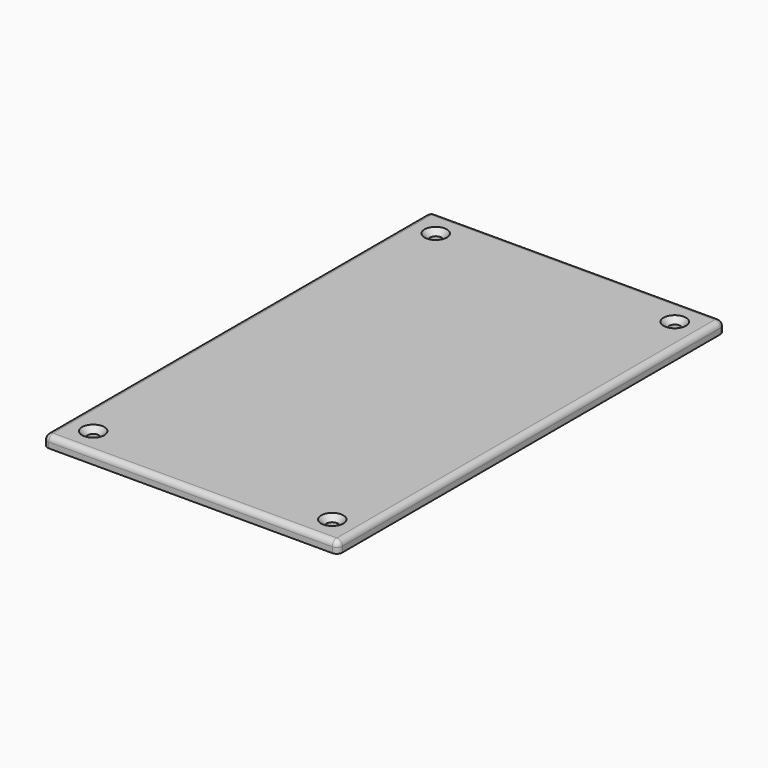
from build123d import *

# Parameters (mm, degrees)
F0_W           = 106
F0_H           = 174
F1_DEPTH       = 4
F2_R           = 2
F3_T1_DEPTH    = 7
F3_S5_W        = 2
F3_S5_H        = 2
F3_T6_DEPTH    = 2
F3_S11_W       = 2
F3_S11_H       = 2
F3_T12_DEPTH   = 2
F3_S17_W       = 2
F3_S17_H       = 2
F3_T18_DEPTH   = 2
F3_S23_W       = 2
F3_S23_H       = 2
F3_T24_DEPTH   = 2
F5_D           = 4.1
F5_DEPTH       = 40
F5_CSINK_D     = 8
F5_CSINK_ANGLE = 90
F5_TIP         = 1.231764269


# Not quite as in the source:
# - a fillet or chamfer that OpenCascade refuses, or shapes differently, is made with other operations: its cross-section is extruded or revolved along the edge and cut away or added


with BuildPart() as f1:
    # F0 (on Top) → F1 (new body)
    with BuildSketch(Plane.XY):
        with Locations((53, 87)):
            Rectangle(F0_W, F0_H)
    extrude(amount=F1_DEPTH)

    # F2
    f2_edges = [f1.edges().sort_by_distance(p)[0] for p in [
        (53, 0, 4),
        (0, 87, 4),
        (106, 87, 4),
        (53, 174, 4),
    ]]
    fillet(f2_edges, radius=F2_R)

    # F3: fillet of radius 2 on 4 edges, made by hand

    # F3_s2 → F3_t1 (cut)
    with BuildSketch(Plane.XY.offset(-5)):
        with BuildLine():
            ThreePointArc((104, 0), (105.4142135624, 0.5857864376), (106, 2))
            Line((106, 2), (106, 0))
            Line((106, 0), (104, 0))
        make_face()
        with BuildLine():
            ThreePointArc((0, 2), (0.5857864376, 0.5857864376), (2, 0))
            Line((2, 0), (0, 0))
            Line((0, 0), (0, 2))
        make_face()
        with BuildLine():
            ThreePointArc((0, 172), (0.5857864376, 173.4142135624), (2, 174))
            Line((2, 174), (0, 174))
            Line((0, 174), (0, 172))
        make_face()
        with BuildLine():
            ThreePointArc((104, 174), (105.4142135624, 173.4142135624), (106, 172))
            Line((106, 172), (106, 174))
            Line((106, 174), (104, 174))
        make_face()
    extrude(amount=F3_T1_DEPTH, mode=Mode.SUBTRACT)


with BuildPart() as f3_tool4:
    # F3_s5 → F3_t6 (new body)
    with BuildSketch(Plane.XZ.offset(-172)):
        with Locations((105, 3)):
            Rectangle(F3_S5_W, F3_S5_H)
    extrude(amount=-F3_T6_DEPTH)

    # F3_s7 → F3_t8 (revolve, cut)
    with BuildSketch(Plane(origin=(104, 172, 2), x_dir=(-0.7071067812, 0, -0.7071067812), z_dir=(0.7071067812, 0, -0.7071067812))):
        with BuildLine():
            ThreePointArc((0, -2), (2, 0), (0, 2))
            Line((0, 2), (0, -2))
        make_face()
    revolve(axis=Axis((104, 172, 2), (0, 1, 0)), mode=Mode.SUBTRACT)


with BuildPart() as f1_1:
    add(f1.part)

    # F3_t3: cut F3_tool4
    add(f3_tool4.part, mode=Mode.SUBTRACT)


with BuildPart() as f3_tool10:
    # F3_s11 → F3_t12 (new body)
    with BuildSketch(Plane.YZ.offset(2)):
        with Locations((173, 3)):
            Rectangle(F3_S11_W, F3_S11_H)
    extrude(amount=-F3_T12_DEPTH)

    # F3_s13 → F3_t14 (revolve, cut)
    with BuildSketch(Plane(origin=(2, 172, 2), x_dir=(0, -0.7071067812, -0.7071067812), z_dir=(0, 0.7071067812, -0.7071067812))):
        with BuildLine():
            ThreePointArc((0, -2), (2, 0), (0, 2))
            Line((0, 2), (0, -2))
        make_face()
    revolve(axis=Axis((2, 172, 2), (-1, 0, 0)), mode=Mode.SUBTRACT)


with BuildPart() as f1_2:
    add(f1_1.part)

    # F3_t9: cut F3_tool10
    add(f3_tool10.part, mode=Mode.SUBTRACT)


with BuildPart() as f3_tool16:
    # F3_s17 → F3_t18 (new body)
    with BuildSketch(Plane.YZ.offset(2)):
        with Locations((1, 3)):
            Rectangle(F3_S17_W, F3_S17_H)
    extrude(amount=-F3_T18_DEPTH)

    # F3_s19 → F3_t20 (revolve, cut)
    with BuildSketch(Plane(origin=(2, 2, 2), x_dir=(0, 0.7071067812, -0.7071067812), z_dir=(0, 0.7071067812, 0.7071067812))):
        with BuildLine():
            ThreePointArc((0, -2), (2, 0), (0, 2))
            Line((0, 2), (0, -2))
        make_face()
    revolve(axis=Axis((2, 2, 2), (-1, 0, 0)), mode=Mode.SUBTRACT)


with BuildPart() as f1_3:
    add(f1_2.part)

    # F3_t15: cut F3_tool16
    add(f3_tool16.part, mode=Mode.SUBTRACT)


with BuildPart() as f3_tool22:
    # F3_s23 → F3_t24 (new body)
    with BuildSketch(Plane.XZ.offset(-2)):
        with Locations((105, 3)):
            Rectangle(F3_S23_W, F3_S23_H)
    extrude(amount=F3_T24_DEPTH)

    # F3_s25 → F3_t26 (revolve, cut)
    with BuildSketch(Plane(origin=(104, 2, 2), x_dir=(-0.7071067812, 0, -0.7071067812), z_dir=(-0.7071067812, 0, 0.7071067812))):
        with BuildLine():
            ThreePointArc((0, -2), (2, 0), (0, 2))
            Line((0, 2), (0, -2))
        make_face()
    revolve(axis=Axis((104, 2, 2), (0, -1, 0)), mode=Mode.SUBTRACT)


with BuildPart() as f1_4:
    add(f1_3.part)

    # F3_t21: cut F3_tool22
    add(f3_tool22.part, mode=Mode.SUBTRACT)

    # F5
    with Locations(Plane.XY.offset(4)):
        with Locations((10, 164), (10, 10), (96, 164), (96, 10)):
            CounterSinkHole(F5_D / 2, F5_CSINK_D / 2, depth=F5_DEPTH, counter_sink_angle=F5_CSINK_ANGLE)
            with Locations((0, 0, -(F5_DEPTH + F5_TIP / 2))):  # 118° drill point
                Cone(0, F5_D / 2, F5_TIP, mode=Mode.SUBTRACT)


solid = f1_4.part
